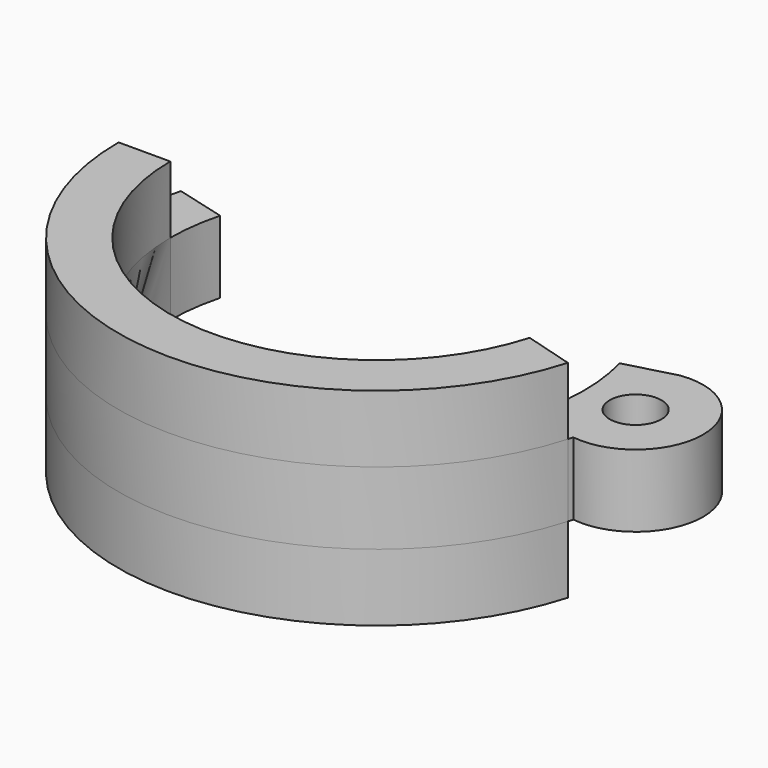
from build123d import *
from build123d import SkipClean  # not in build123d's __all__

# Parameters (mm, degrees)
F1_DEPTH      = 3.5
F2_R          = 1.25
F3_DEPTH      = 3.5
F5_DEPTH      = 3.25
F5_DEPTH_BACK = 6.75


# Not quite as in the source:
# - after a boolean that leaves OpenCascade's solid faulty, fix() repairs it


with BuildPart() as f1:
    # F0 (on Top) → F1 (new body)
    with BuildSketch(Plane.XY):
        with BuildLine():
            ThreePointArc((9.6592582629, 2.588190451), (0, -10), (-9.6592582629, 2.588190451))
            Line((-9.6592582629, 2.588190451), (-12.0740728286, 3.2352380638))
            ThreePointArc((-12.0740728286, 3.2352380638), (-3.2352380638, -12.0740728286), (12.0740728286, -3.2352380638))
            ThreePointArc((12.0740728286, -3.2352380638), (12.5, 0), (12.0740728286, 3.2352380638))
            Line((12.0740728286, 3.2352380638), (9.6592582629, 2.588190451))
        make_face()
        with BuildLine():
            ThreePointArc((12.0740728286, -3.2352380638), (15.7631548055, 0), (12.0740728286, 3.2352380638))
            ThreePointArc((12.0740728286, 3.2352380638), (12.5, 0), (12.0740728286, -3.2352380638))
        make_face()
    extrude(amount=F1_DEPTH)

    # F2 (on face) → F3 (cut, through all)
    with BuildSketch(Plane.XY.offset(3.5)):
        with Locations((12.5, 0)):
            Circle(F2_R)
    extrude(amount=-F3_DEPTH, mode=Mode.SUBTRACT)

    # F4 (on face) → F5 (join, two sides)
    with BuildSketch(Plane(origin=(0, 0, 0), x_dir=(1, 0, 0), z_dir=(0, 0, -1))) as f5_sk:
        with BuildLine():
            ThreePointArc((12.0063097325, 3.4782936344), (-1.7565774028, 12.3759620163), (-12.5, 0))
            Line((-12.5, 0), (-10, 0))
            ThreePointArc((-10, 0), (-1.4052619222, 9.900769613), (9.605047786, 2.7826349075))
            Line((9.605047786, 2.7826349075), (12.0063097325, 3.4782936344))
        make_face()
    with SkipClean():  # cleaning this boolean's faces spoils the solid; the shape is the same uncleaned
        extrude(amount=F5_DEPTH)
        extrude(f5_sk.sketch, amount=-F5_DEPTH_BACK)

    # F6 (on face) → F7 (revolve, cut)
    with BuildSketch(Plane(origin=(0, 0, 0), x_dir=(1, 0, 0), z_dir=(0, 0, -1))):
        with BuildLine():
            Line((-10.9930696768, -1.9515795594), (-11.123595869, -0.960134698))
            ThreePointArc((-11.123595869, -0.960134698), (-11.5540552036, -1.5211202248), (-10.9930696768, -1.9515795594))
        make_face()
    revolve(axis=Axis((-11.0583327729, 1.4558571287, 0), (-0.1305261922, -0.9914448614, 0)), mode=Mode.SUBTRACT)

    add(f1.part.fix(), mode=Mode.REPLACE)


solid = f1.part
